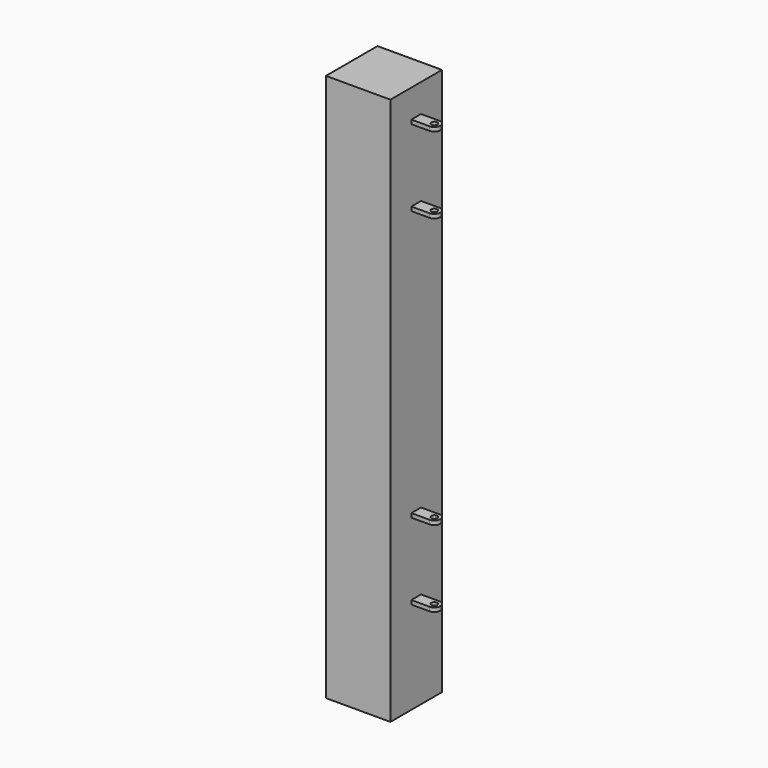
from build123d import *

# Parameters (mm, degrees)
F0_W     = 203.2
F0_H     = 1727.2
F1_DEPTH = 101.6
F2_W     = 38.1
F2_H     = 12.7
F3_DEPTH = 76.2
F4_R     = 19.04999
F5_R     = 9.525
F6_DEPTH = 1638.301


# Not quite as in the source:
# - a fillet or chamfer is up to 0.001 mm smaller than in the source, because OpenCascade refuses the exact size


with BuildPart() as f1:
    # F0 (on Front) → F1 (new body, symmetric)
    with BuildSketch(Plane.XZ):
        Rectangle(F0_W, F0_H)
    extrude(amount=F1_DEPTH, both=True)

    # F2 (on face) → F3 (join)
    with BuildSketch(Plane.YZ.offset(101.6)):
        with Locations((0, -565.15)):
            Rectangle(F2_W, F2_H)
        with Locations((0, -323.85)):
            Rectangle(F2_W, F2_H)
        with Locations((0, 527.05)):
            Rectangle(F2_W, F2_H)
        with Locations((0, 768.35)):
            Rectangle(F2_W, F2_H)
    extrude(amount=F3_DEPTH)

    # F4 (radius 19.05 in the source; OpenCascade refuses exactly that, so slightly less here)
    f4_edges = [f1.edges().sort_by_distance(p)[0] for p in [
        (177.8, 19.05, -565.15),
        (177.8, -19.05, -565.15),
        (177.8, 19.05, -323.85),
        (177.8, -19.05, -323.85),
        (177.8, 19.05, 527.05),
        (177.8, -19.05, 527.05),
        (177.8, 19.05, 768.35),
        (177.8, -19.05, 768.35),
    ]]
    fillet(f4_edges, radius=F4_R)

    # F5 (on face) → F6 (cut, through all)
    with BuildSketch(Plane.XY.offset(774.7)):
        with Locations((158.75, 0)):
            Circle(F5_R)
    extrude(amount=-F6_DEPTH, mode=Mode.SUBTRACT)


solid = f1.part
